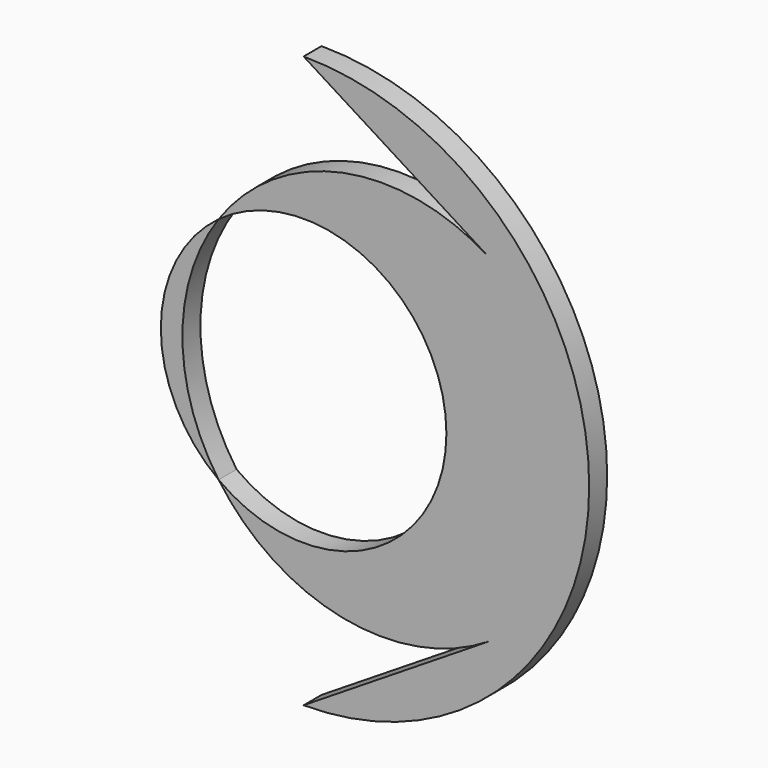
from build123d import *

# Parameters (mm, degrees)
F1_DEPTH = 10


with BuildPart() as f1:
    # F0 (on Front) → F1 (new body)
    with BuildSketch(Plane.XZ):
        with BuildLine():
            ThreePointArc((0, -127), (89.8025612107, -89.8025612107), (127, 0))
            ThreePointArc((127, 0), (89.8025612107, 89.8025612107), (0, 127))
            Line((0, 127), (82.3076020381, 75.2675281207))
            ThreePointArc((82.3076020381, 75.2675281207), (112.8102044117, 42.9974660812), (123.9, 0))
            ThreePointArc((123.9, 0), (112.8102044117, -42.9974660812), (82.3076020381, -75.2675281207))
            Line((82.3076020381, -75.2675281207), (0, -127))
        make_face()
        with BuildLine():
            ThreePointArc((123.9, 0), (112.8102044117, 42.9974660812), (82.3076020381, 75.2675281207))
            ThreePointArc((82.3076020381, 75.2675281207), (17.4103746568, 87.1424987035), (-37.7994285714, 51.0240453088))
            ThreePointArc((-37.7994285714, 51.0240453088), (28.5655936899, 56.7120521331), (63.5, 0))
            ThreePointArc((63.5, 0), (28.5655936899, -56.7120521331), (-37.7994285714, -51.0240453088))
            ThreePointArc((-37.7994285714, -51.0240453088), (17.4103746568, -87.1424987035), (82.3076020381, -75.2675281207))
            ThreePointArc((82.3076020381, -75.2675281207), (112.8102044117, -42.9974660812), (123.9, 0))
        make_face()
    extrude(amount=-F1_DEPTH)


with BuildPart() as f1b:
    # F0 (on Front) → F1, piece 2 (new body)
    with BuildSketch(Plane.XZ):
        with BuildLine():
            ThreePointArc((-37.7994285714, -51.0240453088), (-53.9, 0), (-37.7994285714, 51.0240453088))
            ThreePointArc((-37.7994285714, 51.0240453088), (-63.5, 0), (-37.7994285714, -51.0240453088))
        make_face()
    extrude(amount=-F1_DEPTH)


solid = Compound([f1.part, f1b.part])
